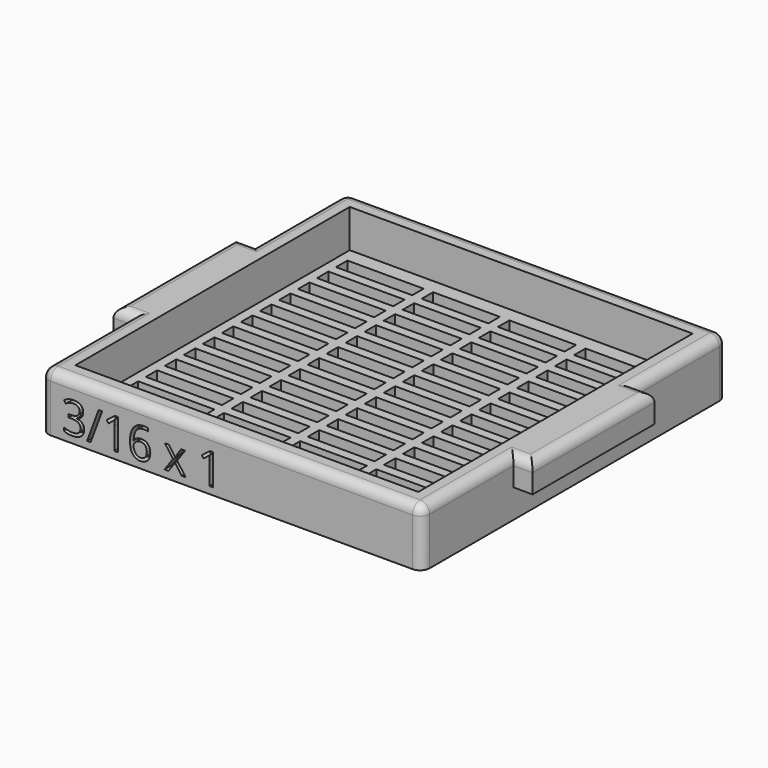
from build123d import *

# Parameters (mm, degrees)
F1_DEPTH     = 6.35
F0_W         = 6.35
F0_H         = 50.8
F2_DEPTH     = 19.05
F3_W         = 25.4
F3_H         = 4.7498
F3_W_2       = 22.225
F4_DEPTH     = 25.4
F5_R         = 3.175
F6_W         = 6.35
F6_H         = 50.8
F7_DEPTH     = 9.525
F8_TEXT_SIZE = 14.4969118992
F9_DEPTH     = 3.175


# Not quite as in the source:
# - a feature names something its author has since deleted; it is built from what else it names
# - Text() gives the source's letters only with a copy of the font that has no kerning and outlines rounded to 1/6400 em; it was checked with that copy


with BuildPart() as f1:
    # F0 (on Top) → F1 (new body)
    with BuildSketch(Plane.XY):
        Polygon((-57.15, 25.1415750563), (-57.15, -25.6584249437), (-57.15, -57.4084249437), (57.15, -57.4084249437), (57.15, -25.6584249437), (57.15, 25.1415750563), (57.15, 56.8915750563), (-57.15, 56.8915750563), align=None)
    extrude(amount=F1_DEPTH)

    # F0 (on Top) → F2 (join)
    with BuildSketch(Plane.XY):
        Polygon((-63.5, -25.6584249437), (-63.5, -63.7584249437), (63.5, -63.7584249437), (63.5, -25.6584249437), (57.15, -25.6584249437), (57.15, -57.4084249437), (-57.15, -57.4084249437), (-57.15, -25.6584249437), align=None)
        with Locations((-66.675, -0.2584249437)):
            Rectangle(F0_W, F0_H)
        with Locations((-60.325, -0.2584249437)):
            Rectangle(F0_W, F0_H)
        with Locations((60.325, -0.2584249437)):
            Rectangle(F0_W, F0_H)
        with Locations((66.675, -0.2584249437)):
            Rectangle(F0_W, F0_H)
        Polygon((-63.5, 63.2415750563), (-63.5, 25.1415750563), (-57.15, 25.1415750563), (-57.15, 56.8915750563), (57.15, 56.8915750563), (57.15, 25.1415750563), (63.5, 25.1415750563), (63.5, 63.2415750563), align=None)
    extrude(amount=F2_DEPTH)

    # F3 (on face) → F4 (cut)
    with BuildSketch(Plane.XY.offset(6.35)):
        with Locations((-41.275, -45.5085249437)):
            Rectangle(F3_W, F3_H)
        with Locations((-41.275, -37.5837249437)):
            Rectangle(F3_W, F3_H)
        with Locations((-41.275, -29.6589249437)):
            Rectangle(F3_W, F3_H)
        with Locations((-41.275, -21.7341249437)):
            Rectangle(F3_W, F3_H)
        with Locations((-41.275, -13.8093249437)):
            Rectangle(F3_W, F3_H)
        with Locations((-41.275, -5.8845249437)):
            Rectangle(F3_W, F3_H)
        with Locations((-41.275, 2.0402750563)):
            Rectangle(F3_W, F3_H)
        with Locations((-41.275, 9.9650750563)):
            Rectangle(F3_W, F3_H)
        with Locations((-41.275, 17.8898750563)):
            Rectangle(F3_W, F3_H)
        with Locations((-41.275, 25.8146750563)):
            Rectangle(F3_W, F3_H)
        with Locations((-41.275, 33.7394750563)):
            Rectangle(F3_W, F3_H)
        with Locations((-41.275, 41.6642750563)):
            Rectangle(F3_W, F3_H)
        with Locations((-41.275, 49.5890750563)):
            Rectangle(F3_W, F3_H)
        with Locations((-14.2875, -45.5085249437)):
            Rectangle(F3_W_2, F3_H)
        with Locations((-14.2875, -37.5837249437)):
            Rectangle(F3_W_2, F3_H)
        with Locations((11.1125, -45.5085249437)):
            Rectangle(F3_W_2, F3_H)
        with Locations((11.1125, -37.5837249437)):
            Rectangle(F3_W_2, F3_H)
        with Locations((38.1, -45.5085249437)):
            Rectangle(F3_W, F3_H)
        with Locations((38.1, -37.5837249437)):
            Rectangle(F3_W, F3_H)
        with Locations((38.1, -29.6589249437)):
            Rectangle(F3_W, F3_H)
        with Locations((38.1, -21.7341249437)):
            Rectangle(F3_W, F3_H)
        with Locations((11.1125, -21.7341249437)):
            Rectangle(F3_W_2, F3_H)
        with Locations((11.1125, -29.6589249437)):
            Rectangle(F3_W_2, F3_H)
        with Locations((-14.2875, -29.6589249437)):
            Rectangle(F3_W_2, F3_H)
        with Locations((-14.2875, -21.7341249437)):
            Rectangle(F3_W_2, F3_H)
        with Locations((38.1, -13.8093249437)):
            Rectangle(F3_W, F3_H)
        with Locations((38.1, -5.8845249437)):
            Rectangle(F3_W, F3_H)
        with Locations((38.1, 2.0402750563)):
            Rectangle(F3_W, F3_H)
        with Locations((11.1125, -13.8093249437)):
            Rectangle(F3_W_2, F3_H)
        with Locations((11.1125, -5.8845249437)):
            Rectangle(F3_W_2, F3_H)
        with Locations((11.1125, 2.0402750563)):
            Rectangle(F3_W_2, F3_H)
        with Locations((-14.2875, -13.8093249437)):
            Rectangle(F3_W_2, F3_H)
        with Locations((-14.2875, -5.8845249437)):
            Rectangle(F3_W_2, F3_H)
        with Locations((-14.2875, 2.0402750563)):
            Rectangle(F3_W_2, F3_H)
        with Locations((-14.2875, 9.9650750563)):
            Rectangle(F3_W_2, F3_H)
        with Locations((-14.2875, 17.8898750563)):
            Rectangle(F3_W_2, F3_H)
        with Locations((-14.2875, 25.8146750563)):
            Rectangle(F3_W_2, F3_H)
        with Locations((-14.2875, 33.7394750563)):
            Rectangle(F3_W_2, F3_H)
        with Locations((11.1125, 9.9650750563)):
            Rectangle(F3_W_2, F3_H)
        with Locations((11.1125, 17.8898750563)):
            Rectangle(F3_W_2, F3_H)
        with Locations((11.1125, 25.8146750563)):
            Rectangle(F3_W_2, F3_H)
        with Locations((11.1125, 33.7394750563)):
            Rectangle(F3_W_2, F3_H)
        with Locations((38.1, 33.7394750563)):
            Rectangle(F3_W, F3_H)
        with Locations((38.1, 25.8146750563)):
            Rectangle(F3_W, F3_H)
        with Locations((38.1, 17.8898750563)):
            Rectangle(F3_W, F3_H)
        with Locations((38.1, 9.9650750563)):
            Rectangle(F3_W, F3_H)
        with Locations((-14.2875, 41.6642750563)):
            Rectangle(F3_W_2, F3_H)
        with Locations((-14.2875, 49.5890750563)):
            Rectangle(F3_W_2, F3_H)
        with Locations((11.1125, 49.5890750563)):
            Rectangle(F3_W_2, F3_H)
        with Locations((11.1125, 41.6642750563)):
            Rectangle(F3_W_2, F3_H)
        with Locations((38.1, 41.6642750563)):
            Rectangle(F3_W, F3_H)
        with Locations((38.1, 49.5890750563)):
            Rectangle(F3_W, F3_H)
    extrude(amount=-F4_DEPTH, mode=Mode.SUBTRACT)

    # F5
    f5_edges = [f1.edges().sort_by_distance(p)[0] for p in [
        (-63.5, -44.708425, 19.05),
        (0, -63.758425, 19.05),
        (63.5, -44.708425, 19.05),
        (66.675, -25.658425, 19.05),
        (69.85, -0.258425, 19.05),
        (-66.675, -25.658425, 19.05),
        (-69.85, -0.258425, 19.05),
        (-66.675, 25.141575, 19.05),
        (-63.5, 44.191575, 19.05),
        (0, 63.241575, 19.05),
        (63.5, 44.191575, 19.05),
        (66.675, 25.141575, 19.05),
        (63.5, -63.758425, 9.525),
        (-63.5, -63.758425, 9.525),
        (-63.5, 63.241575, 9.525),
        (63.5, 63.241575, 9.525),
    ]]
    fillet(f5_edges, radius=F5_R)

    # F6 (on face) → F7 (cut)
    with BuildSketch(Plane(origin=(0, 0, 0), x_dir=(1, 0, 0), z_dir=(0, 0, -1))):
        with Locations((-66.675, 0.2584249437)):
            Rectangle(F6_W, F6_H)
        with Locations((66.675, 0.2584249437)):
            Rectangle(F6_W, F6_H)
    extrude(amount=-F7_DEPTH, mode=Mode.SUBTRACT)

    # F8 (on face) → F9 (cut)
    with BuildSketch(Plane.XZ.offset(63.7584249437)):
        with Locations((-56.5979406238, 2.3586850148)):
            Text('3/16 x 1', F8_TEXT_SIZE, font='Open Sans', text_align=(TextAlign.LEFT, TextAlign.BOTTOM))
    extrude(amount=-F9_DEPTH, mode=Mode.SUBTRACT)


solid = f1.part
